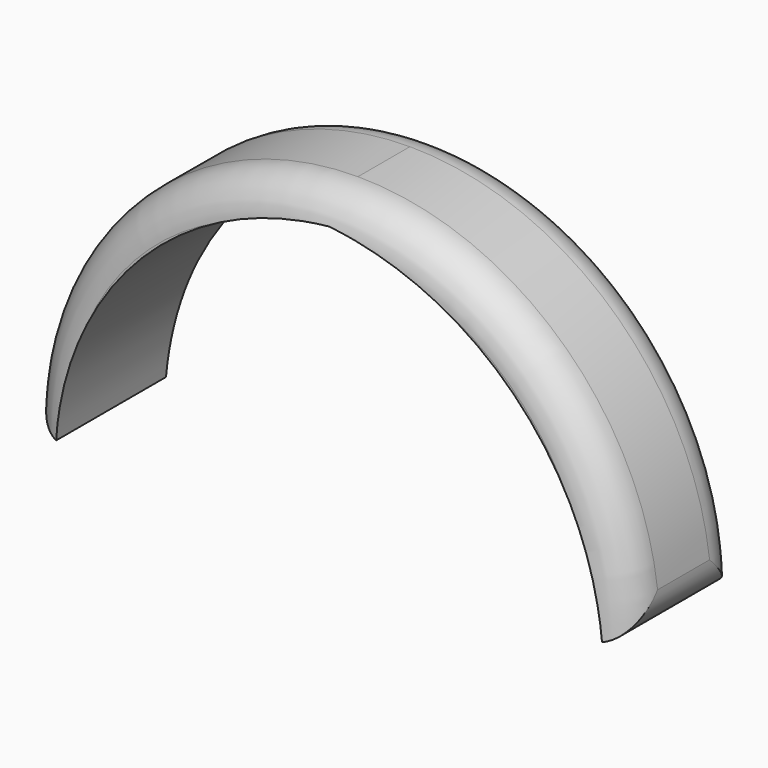
from build123d import *

# Parameters (mm, degrees)
F1_DEPTH    = 19.05
F2_T1_DEPTH = 46.4897133591
F2_T4_ANGLE = 217.0620929047
F2_T6_ANGLE = 217.0620929047


# Not quite as in the source:
# - a fillet or chamfer that OpenCascade refuses, or shapes differently, is made with other operations: its cross-section is extruded or revolved along the edge and cut away or added


with BuildPart() as f1:
    # F0 (on Front) → F1 (new body)
    with BuildSketch(Plane.XZ):
        with BuildLine():
            Line((37.3471569497, 8.89), (41.275, 8.89))
            ThreePointArc((41.275, 8.89), (29.4111956787, 38.4857608957), (0, 50.8))
            ThreePointArc((0, 50.8), (-29.4111956787, 38.4857608957), (-41.275, 8.89))
            Line((-41.275, 8.89), (-37.3471569497, 8.89))
            ThreePointArc((-37.3471569497, 8.89), (-25.6019859935, 34.6749584003), (0, 46.8137982826))
            ThreePointArc((0, 46.8137982826), (25.6019859935, 34.6749584003), (37.3471569497, 8.89))
        make_face()
    extrude(amount=F1_DEPTH)

    # F2: fillet of radius 5.08 on 4 edges, made by hand

    # F2_s2 → F2_t1 (cut)
    with BuildSketch(Plane.XZ.offset(-13.7198566795)):
        with BuildLine():
            ThreePointArc((40.9938405607, 14.3707357297), (40.1783895926, 10.9597537028), (37.3471569497, 8.89))
            Line((37.3471569497, 8.89), (41.275, 8.89))
            ThreePointArc((41.275, 8.89), (41.2256006364, 11.6350453788), (40.9938405607, 14.3707357297))
        make_face()
        with BuildLine():
            ThreePointArc((-37.3471569497, 8.89), (-40.1783895926, 10.9597537028), (-40.9938405607, 14.3707357297))
            ThreePointArc((-40.9938405607, 14.3707357297), (-41.2256006364, 11.6350453788), (-41.275, 8.89))
            Line((-41.275, 8.89), (-37.3471569497, 8.89))
        make_face()
    extrude(amount=F2_T1_DEPTH, mode=Mode.SUBTRACT)

    # F2_s3 → F2_t4 (revolve, cut)
    with BuildSketch(Plane(origin=(2.8688146876, 0, 8.5585685763), x_dir=(0, 1, 0), z_dir=(-0.3178184711, 0, -0.9481515804))):
        with BuildLine():
            ThreePointArc((-5.08, 38.2541185681), (-1.4878975516, 36.7662210165), (0, 33.1741185681))
            Line((0, 33.1741185681), (0, 38.2541185681))
            Line((0, 38.2541185681), (-5.08, 38.2541185681))
        make_face()
    revolve(axis=Axis((0, 0, 9.5201893939), (0, -1, 0)), revolution_arc=F2_T4_ANGLE, mode=Mode.SUBTRACT)

    # F2_s5 → F2_t6 (revolve, cut)
    with BuildSketch(Plane(origin=(-2.8688146876, 0, 8.5585685763), x_dir=(0, 1, 0), z_dir=(0.3178184711, 0, -0.9481515804))):
        with BuildLine():
            ThreePointArc((-19.05, -33.1741185681), (-17.5621024484, -36.7662210165), (-13.97, -38.2541185681))
            Line((-13.97, -38.2541185681), (-19.05, -38.2541185681))
            Line((-19.05, -38.2541185681), (-19.05, -33.1741185681))
        make_face()
    revolve(axis=Axis((0, -19.05, 9.5201893939), (0, 1, 0)), revolution_arc=F2_T6_ANGLE, mode=Mode.SUBTRACT)


solid = f1.part
